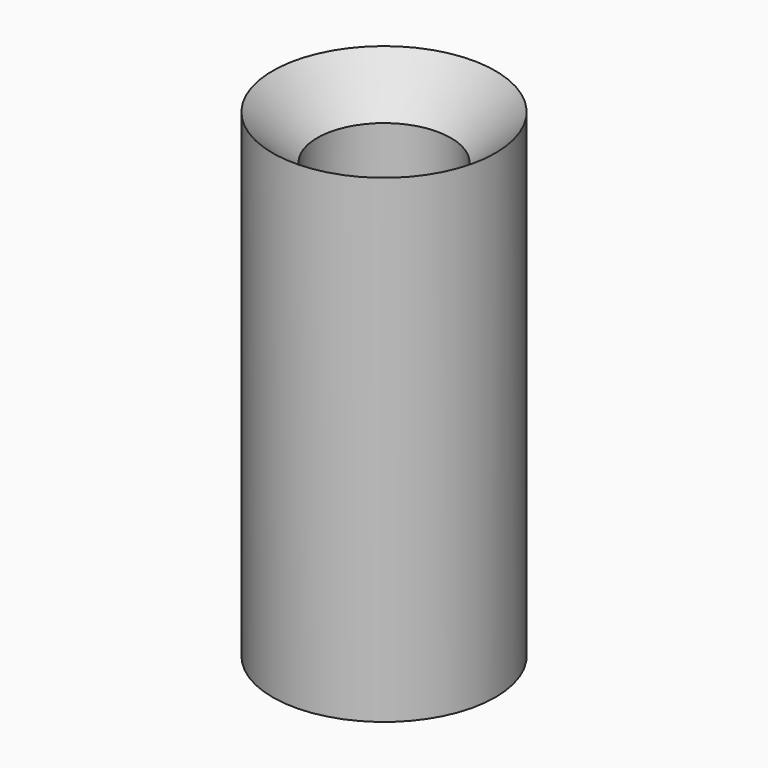
from build123d import *

# Parameters (mm, degrees)
F0_R     = 20
F1_DEPTH = 86
F2_T     = -8
F3_SIZE  = 7.99999


# Not quite as in the source:
# - a fillet or chamfer is up to 0.001 mm smaller than in the source, because OpenCascade refuses the exact size


with BuildPart() as f1:
    # F0 (on Top) → F1 (new body)
    with BuildSketch(Plane.XY):
        Circle(F0_R)
    extrude(amount=F1_DEPTH)

    # F2
    f2_openings = [f1.faces().sort_by_distance(p)[0] for p in [
        (0, 0, 86),
    ]]
    offset(amount=F2_T, openings=f2_openings)

    # F3 (size 8 in the source; OpenCascade refuses exactly that, so slightly less here)
    f3_edges = [f1.edges().sort_by_distance(p)[0] for p in [
        (-12, 0, 86),
    ]]
    chamfer(f3_edges, length=F3_SIZE)


solid = f1.part
